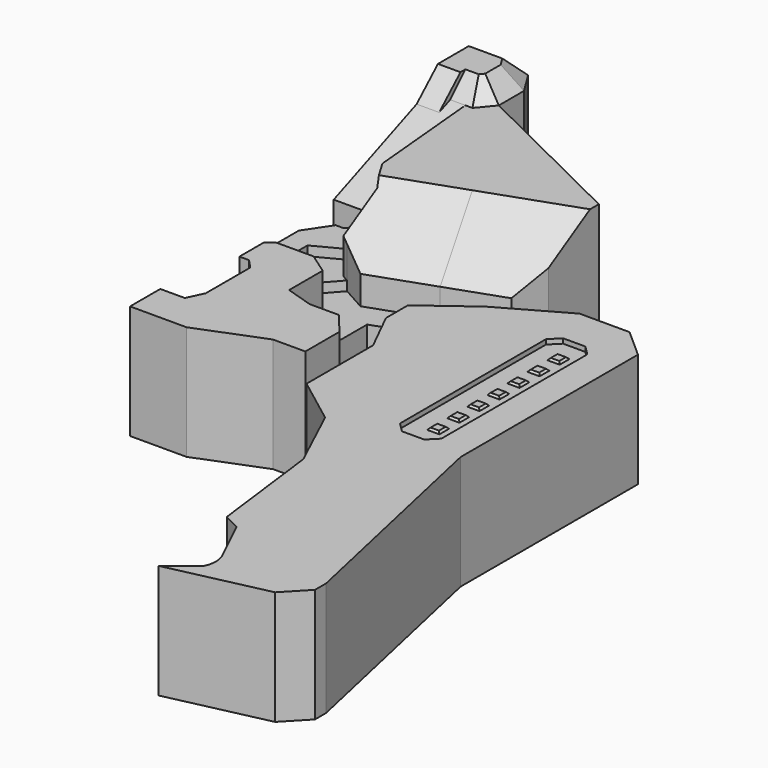
from build123d import *

# Parameters (mm, degrees)
F1_DEPTH  = 3.175
F2_DEPTH  = 0.635
F3_DEPTH  = 0.9525
F4_DEPTH  = 1.27
F5_DEPTH  = 0.9525
F6_DEPTH  = 1.905
F7_DEPTH  = 1.905
F8_SIZE2  = 3.920404
F8_SIZE   = 1.58749
F9_DEPTH  = 3.175
F10_SIZE2 = 2.54
F10_SIZE  = 1.5875
F0_W      = 0.4064
F0_H      = 0.4064
F11_DEPTH = 1.74625
F12_DEPTH = 1.80975
F13_SIZE  = 0.06349
F14_DEPTH = 3.81
F15_SIZE  = 0.635
F16_SIZE2 = 0.889
F16_SIZE  = 0.82169


# Not quite as in the source:
# - a fillet or chamfer is up to 0.001 mm smaller than in the source, because OpenCascade refuses the exact size


with BuildPart() as f1:
    # F0 (on Top) → F1 (new body, symmetric)
    with BuildSketch(Plane.XY):
        Polygon((-50.6281256676, 71.2183639407), (-50.6281256676, 70.1812039194), (-49.8182103038, 70.1812039194), (-49.8182103038, 70.8826556802), (-50.1483604312, 71.2183639407), align=None)
        Polygon((-50.1740800176, 73.6415099857), (-50.9259268409, 73.6415099857), (-50.9259268409, 70.1812039194), (-50.6281256676, 70.1812039194), (-50.6281256676, 71.2183639407), (-50.1483604312, 71.2183639407), (-49.8182103038, 70.8826556802), (-49.8182103038, 70.1812039194), (-49.3029352417, 70.1812039194), (-49.6676526964, 74.1016089545), (-50.1740800176, 74.1016089545), align=None)
    extrude(amount=F1_DEPTH, both=True)

    # F0 (on Top) → F4 (join, symmetric)
    with BuildSketch(Plane.XY):
        Polygon((-50.3666736186, 69.5621669292), (-50.9259268409, 68.7222108245), (-50.9259268409, 66.6679893427), (-50.4561580682, 66.6679893427), (-50.2266827847, 66.8746345481), (-50.2266827847, 68.2110610151), (-48.7899799626, 68.9663514404), (-48.7899799626, 69.3257788249), (-49.3029352417, 70.1812039194), (-49.8182103038, 70.1812039194), (-49.8182103038, 69.8665380478), (-50.1052215695, 69.5621669292), align=None)
    extrude(amount=F4_DEPTH, both=True)

    # F0 (on Top) → F5 (join, symmetric)
    with BuildSketch(Plane.XY):
        Polygon((-50.4561580682, 66.6679893427), (-50.9259268409, 66.6679893427), (-50.9259268409, 62.9424099233), (-50.1054741972, 62.9424099233), (-49.8480494991, 63.4934638042), (-49.8480494991, 65.3477449007), (-50.1348926713, 65.6577164373), (-50.4561580682, 65.6577164373), align=None)
    extrude(amount=F5_DEPTH, both=True)

    # F0 (on Top) → F6 (join, symmetric)
    with BuildSketch(Plane.XY):
        Polygon((-50.1054741972, 62.9424099233), (-50.9259268409, 62.9424099233), (-50.9259268409, 61.6806034717), (-49.9836847533, 61.6806034717), (-49.0414426658, 61.6806034717), (-46.8467983999, 62.5481613564), (-45.7673492018, 62.5481613564), (-45.7673492018, 63.96457699), (-46.3623406364, 64.7048412492), (-46.9843501341, 64.7048412492), (-47.3467745018, 64.7048412492), (-48.2646719072, 64.9918522074), (-48.2646719072, 66.3924624023), (-48.9530977577, 66.8746345481), (-49.3798330426, 66.8746345481), (-50.2266827847, 66.8746345481), (-50.4561580682, 66.6679893427), (-50.4561580682, 65.6577164373), (-50.1348926713, 65.6577164373), (-49.8480494991, 65.3477449007), (-49.8480494991, 63.4934638042), align=None)
    extrude(amount=F6_DEPTH, both=True)

    # F8 (size 1.5875 and 3.9204138 in the source; OpenCascade refuses exactly that, so slightly less here)
    f8_edges = [f1.edges().sort_by_distance(p)[0] for p in [
        (-50.114431, 70.181204, 3.175),
    ]]
    f8_side = f1.faces().sort_by_distance((-50.194999, 70.181204, 0))[0]
    chamfer(f8_edges, length=F8_SIZE, length2=F8_SIZE2, reference=f8_side)


with BuildPart() as f2:
    # F0 (on Top) → F2 (new body, symmetric)
    with BuildSketch(Plane.XY):
        Polygon((-48.5652523943, 67.789411228), (-49.3798330426, 66.8746345481), (-48.9530977577, 66.8746345481), (-48.2646719072, 66.3924624023), (-48.2646719072, 64.9918522074), (-47.3467745018, 64.7048412492), (-46.9843501341, 64.7048412492), (-46.9843501341, 66.647020211), (-46.3370832544, 66.8746345481), (-45.6853446256, 68.0750405093), (-47.7640694044, 67.3440475027), align=None)
    extrude(amount=F2_DEPTH, both=True)


with BuildPart() as f3:
    # F0 (on Top) → F3 (new body, symmetric)
    with BuildSketch(Plane.XY):
        Polygon((-50.2266827847, 68.2110610151), (-50.2266827847, 66.8746345481), (-49.3798330426, 66.8746345481), (-48.5652523943, 67.789411228), (-48.7899799626, 67.9143333847), (-48.7899799626, 68.9663514404), align=None)
    extrude(amount=F3_DEPTH, both=True)


with BuildPart() as f7:
    # F0 (on Top) → F7 (new body, symmetric)
    with BuildSketch(Plane.XY):
        with BuildLine():
            Line((-38.8841607986, 67.8256603618), (-39.7055770052, 68.5543456876))
            Line((-39.7055770052, 68.5543456876), (-39.8507907079, 68.6831660024))
            Line((-39.8507907079, 68.6831660024), (-41.5209472054, 68.6831660024))
            Line((-41.5209472054, 68.6831660024), (-43.6801923594, 67.4623179713))
            Line((-43.6801923594, 67.4623179713), (-45.3071346471, 66.253006158))
            Line((-45.3071346471, 66.253006158), (-45.3071346471, 65.6813332453))
            Line((-45.3071346471, 65.6813332453), (-45.3071346471, 65.3379186988))
            Line((-45.3071346471, 65.3379186988), (-44.6054935455, 63.9231130481))
            Line((-44.6054935455, 63.9231130481), (-44.6054935455, 61.1467398703))
            Line((-44.6054935455, 61.1467398703), (-43.0343933403, 59.9568933249))
            Line((-43.0343933403, 59.9568933249), (-42.0097745955, 57.7639564872))
            Line((-42.0097745955, 57.7639564872), (-41.5328480303, 53.9781488478))
            Line((-41.5328480303, 53.9781488478), (-40.9777127206, 53.693279624))
            Line((-40.9777127206, 53.693279624), (-40.2664281428, 52.2122420371))
            ThreePointArc((-40.2664281428, 52.2122420371), (-40.1788901735, 51.8277678639), (-40.2664281428, 51.4432936907))
            Line((-40.2664281428, 51.4432936907), (-41.2004438284, 50.7033893074))
            Line((-41.2004438284, 50.7033893074), (-37.8901109325, 51.436453213))
            Line((-37.8901109325, 51.436453213), (-37.1640972953, 52.1977802048))
            Line((-37.1640972953, 52.1977802048), (-37.1640972953, 52.6581140739))
            Line((-37.1640972953, 52.6581140739), (-38.8841607986, 60.4254898161))
            Line((-38.8841607986, 60.4254898161), (-38.8841607986, 67.8256603618))
        make_face()
        Polygon((-41.3026166391, 60.9196083232), (-41.3026166391, 67.0101981577), (-40.9848232462, 67.3279915506), (-40.2416022253, 67.3279915506), (-39.9238088324, 67.0101981577), (-39.9238088324, 60.9196083232), (-40.2416022253, 60.6018149303), (-40.9848232462, 60.6018149303), align=None, mode=Mode.SUBTRACT)
    extrude(amount=F7_DEPTH, both=True)

    # F0 (on Top) → F11 (join, symmetric)
    with BuildSketch(Plane.XY):
        Polygon((-40.9848232462, 67.3279915506), (-41.3026166391, 67.0101981577), (-41.3026166391, 60.9196083232), (-40.9848232462, 60.6018149303), (-40.2416022253, 60.6018149303), (-39.9238088324, 60.9196083232), (-39.9238088324, 67.0101981577), (-40.2416022253, 67.3279915506), align=None)
        with Locations((-40.5086720156, 61.5175491821)):
            Rectangle(F0_W, F0_H, mode=Mode.SUBTRACT)
        with Locations((-40.5099353882, 62.35574823)):
            Rectangle(F0_W, F0_H, mode=Mode.SUBTRACT)
        with Locations((-40.5111987609, 63.1939472779)):
            Rectangle(F0_W, F0_H, mode=Mode.SUBTRACT)
        with Locations((-40.5124621335, 64.0321463258)):
            Rectangle(F0_W, F0_H, mode=Mode.SUBTRACT)
        with Locations((-40.5137255062, 64.8703453737)):
            Rectangle(F0_W, F0_H, mode=Mode.SUBTRACT)
        with Locations((-40.5149888788, 65.7085444216)):
            Rectangle(F0_W, F0_H, mode=Mode.SUBTRACT)
        with Locations((-40.5162522515, 66.5467434695)):
            Rectangle(F0_W, F0_H, mode=Mode.SUBTRACT)
    extrude(amount=F11_DEPTH, both=True)

    # F0 (on Top) → F12 (join, symmetric)
    with BuildSketch(Plane.XY):
        with Locations((-40.5162522515, 66.5467434695)):
            Rectangle(F0_W, F0_H)
        with Locations((-40.5149888788, 65.7085444216)):
            Rectangle(F0_W, F0_H)
        with Locations((-40.5137255062, 64.8703453737)):
            Rectangle(F0_W, F0_H)
        with Locations((-40.5124621335, 64.0321463258)):
            Rectangle(F0_W, F0_H)
        with Locations((-40.5111987609, 63.1939472779)):
            Rectangle(F0_W, F0_H)
        with Locations((-40.5099353882, 62.35574823)):
            Rectangle(F0_W, F0_H)
        with Locations((-40.5086720156, 61.5175491821)):
            Rectangle(F0_W, F0_H)
    extrude(amount=F12_DEPTH, both=True)

    # F13 (size 0.0635 in the source; OpenCascade refuses exactly that, so slightly less here)
    f13_edges = [f7.edges().sort_by_distance(p)[0] for p in [
        (-40.305472, 61.517549, 1.80975),
        (-40.508672, 61.314349, 1.80975),
        (-40.516252, 66.749943, 1.80975),
        (-40.719452, 66.546743, 1.80975),
        (-40.516252, 66.343543, 1.80975),
        (-40.313052, 66.546743, 1.80975),
        (-40.514989, 65.911744, 1.80975),
        (-40.718189, 65.708544, 1.80975),
        (-40.514989, 65.505344, 1.80975),
        (-40.311789, 65.708544, 1.80975),
        (-40.513726, 65.073545, 1.80975),
        (-40.716926, 64.870345, 1.80975),
        (-40.513726, 64.667145, 1.80975),
        (-40.310526, 64.870345, 1.80975),
        (-40.512462, 64.235346, 1.80975),
        (-40.715662, 64.032146, 1.80975),
        (-40.512462, 63.828946, 1.80975),
        (-40.309262, 64.032146, 1.80975),
        (-40.511199, 63.397147, 1.80975),
        (-40.714399, 63.193947, 1.80975),
        (-40.511199, 62.990747, 1.80975),
        (-40.307999, 63.193947, 1.80975),
        (-40.509935, 62.558948, 1.80975),
        (-40.713135, 62.355748, 1.80975),
        (-40.509935, 62.152548, 1.80975),
        (-40.306735, 62.355748, 1.80975),
        (-40.508672, 61.720749, 1.80975),
        (-40.711872, 61.517549, 1.80975),
    ]]
    chamfer(f13_edges, length=F13_SIZE)


with BuildPart() as f9:
    # F0 (on Top) → F9 (new body, symmetric)
    with BuildSketch(Plane.XY):
        Polygon((-43.4626820801, 71.9161705457), (-48.9835043047, 74.6411937319), (-49.4308925539, 74.1016089545), (-49.6676526964, 74.1016089545), (-49.3029352417, 70.1812039194), (-48.7899799626, 69.3257788249), (-48.7899799626, 68.9663514404), (-48.7899799626, 67.9143333847), (-48.5652523943, 67.789411228), (-47.7640694044, 67.3440475027), (-45.6853446256, 68.0750405093), (-43.8314122647, 68.7269842416), (-43.4626820801, 69.8105162318), (-43.4626820801, 71.0267184557), align=None)
    extrude(amount=F9_DEPTH, both=True)

    # F10
    f10_edges = [f9.edges().sort_by_distance(p)[0] for p in [
        (-45.797741, 68.035516, 3.175),
    ]]
    f10_side = f9.faces().sort_by_distance((-45.797741, 68.035516, 0))[0]
    chamfer(f10_edges, length=F10_SIZE, length2=F10_SIZE2, reference=f10_side)


with BuildPart() as f14:
    # F0 (on Top) → F14 (new body, symmetric)
    with BuildSketch(Plane.XY):
        Polygon((-49.4530850453, 76.451984704), (-50.9259268409, 76.451984704), (-50.9259268409, 73.6415099857), (-50.1740800176, 73.6415099857), (-50.1740800176, 74.1016089545), (-49.6676526964, 74.1016089545), (-49.4308925539, 74.1016089545), (-48.9835043047, 74.6411937319), (-48.9835043047, 75.6947181328), align=None)
    extrude(amount=F14_DEPTH, both=True)

    # F15
    f15_edges = [f14.edges().sort_by_distance(p)[0] for p in [
        (-49.802486, 74.101609, 3.81),
        (-49.207198, 74.371401, 3.81),
        (-48.983504, 75.167956, 3.81),
        (-49.218295, 76.073351, 3.81),
        (-50.189506, 76.451985, 3.81),
    ]]
    chamfer(f15_edges, length=F15_SIZE)

    # F16
    f16_edges = [f14.edges().sort_by_distance(p)[0] for p in [
        (-50.550003, 73.64151, 3.81),
    ]]
    f16_side = f14.faces().sort_by_distance((-50.550003, 73.64151, 0))[0]
    chamfer(f16_edges, length=F16_SIZE, length2=F16_SIZE2, reference=f16_side)


solid = Compound([f1.part, f2.part, f3.part, f7.part, f9.part, f14.part])
